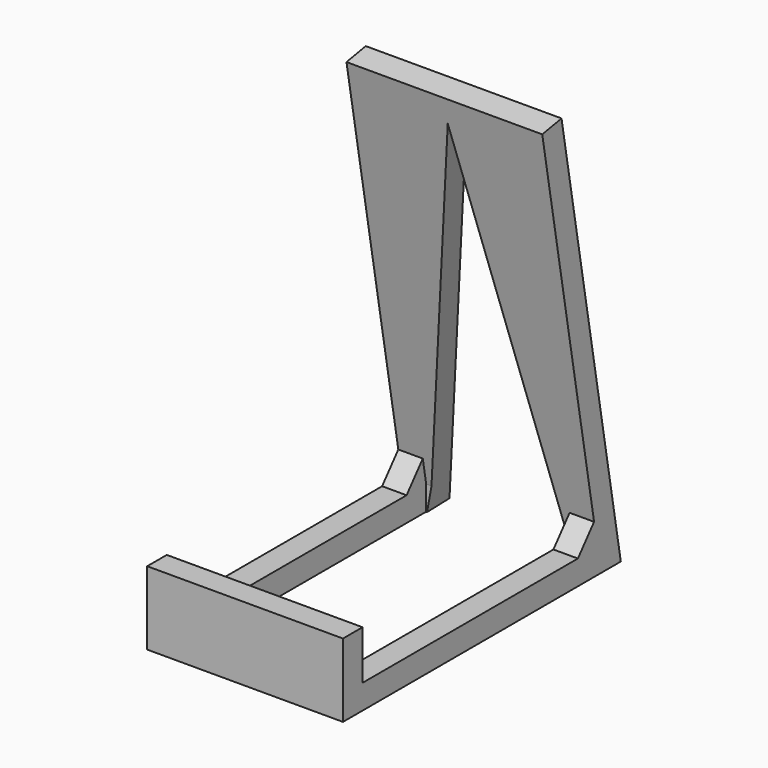
from build123d import *

# Parameters (mm, degrees)
F1_DEPTH    = 50.8
F2_W        = 38.1
F2_H        = 76.2
F3_DEPTH    = 25.4
F5_DEPTH    = 25.4
F6_T1_DEPTH = 6.35
F6_T3_DEPTH = 6.35


# Not quite as in the source:
# - a fillet or chamfer that OpenCascade refuses, or shapes differently, is made with other operations: its cross-section is extruded or revolved along the edge and cut away or added


with BuildPart() as f1:
    # F0 (on Right) → F1 (new body)
    with BuildSketch(Plane.YZ):
        Polygon((36.5886149989, -22.4861702016), (-39.6113850011, -22.4861702016), (-39.6113850011, -9.7861702016), (-45.9613837302, -9.7861702016), (-45.9613837302, -28.8361689307), (44.1562487973, -28.8361689307), (24.927321739, 80.2164955059), (18.673793759, 79.1138297984), align=None)
    extrude(amount=F1_DEPTH)

    # F2 (on face) → F3 (cut)
    with BuildSketch(Plane.XY.offset(-22.4861702016)):
        with Locations((25.4, -1.5113850011)):
            Rectangle(F2_W, F2_H)
    extrude(amount=-F3_DEPTH, mode=Mode.SUBTRACT)

    # F4 (on face) → F5 (cut)
    with BuildSketch(Plane(origin=(0, 37.8934996616, 6.6816463838), x_dir=(-1, 0, 0), z_dir=(0, 0.984807753, 0.1736481777))):
        Polygon((-25.4, 68.3192426996), (-44.45, -36.0657348664), (-6.35, -36.0657348664), align=None)
    extrude(amount=-F5_DEPTH, mode=Mode.SUBTRACT)

    # F6: chamfer of 6.35 on 4 edges, made by hand

    # F6_s2 → F6_t1 (join)
    with BuildSketch(Plane.YZ):
        Polygon((35.4859490708, -16.23264097), (30.2386149989, -22.4861702016), (36.5886149989, -22.4861702016), align=None)
    extrude(amount=F6_T1_DEPTH)

    # F6_s4 → F6_t3 (join)
    with BuildSketch(Plane.YZ.offset(44.45)):
        Polygon((35.4859490708, -16.23264097), (30.2386149989, -22.4861702016), (36.5886149989, -22.4861702016), align=None)
    extrude(amount=F6_T3_DEPTH)


solid = f1.part
